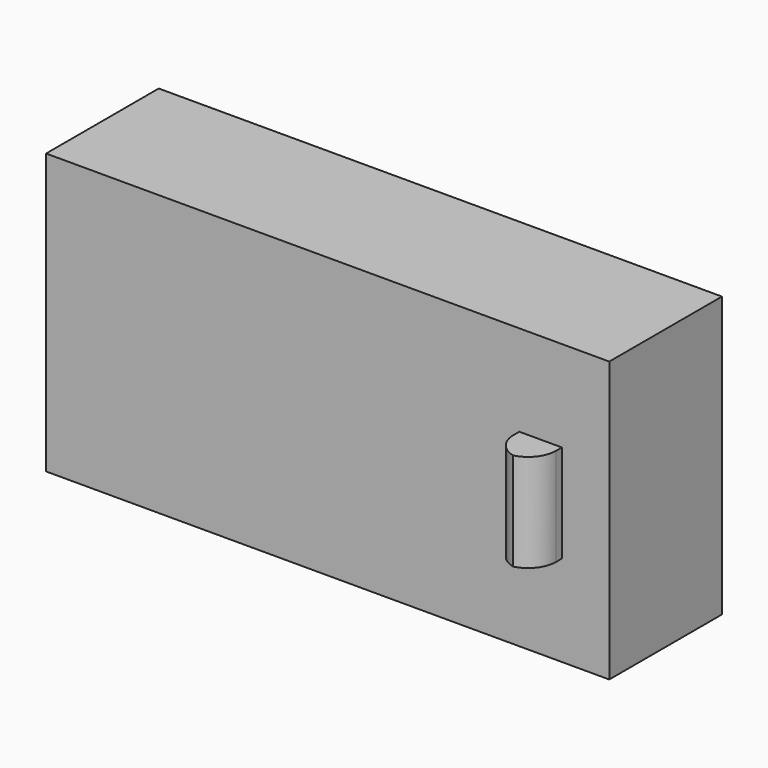
from build123d import *

# Parameters (mm, degrees)
F0_W        = 7.6837688684
F0_H        = 17.6492575556
F1_DEPTH    = 31.75
F0_W_2      = 101.6
F0_H_2      = 50.4952
F2_DEPTH    = 25.4
F3_T1_DEPTH = 43.0492575556


# Not quite as in the source:
# - a fillet or chamfer that OpenCascade refuses, or shapes differently, is made with other operations: its cross-section is extruded or revolved along the edge and cut away or added


with BuildPart() as f1:
    # F0 (on Front) → F1 (new body)
    with BuildSketch(Plane.XZ):
        with Locations((38.4069420397, 0)):
            Rectangle(F0_W, F0_H)
    extrude(amount=F1_DEPTH)

    # F0 (on Front) → F2 (join)
    with BuildSketch(Plane.XZ):
        Rectangle(F0_W_2, F0_H_2)
        with Locations((38.4069420397, 0)):
            Rectangle(F0_W, F0_H, mode=Mode.SUBTRACT)
    extrude(amount=F2_DEPTH)

    # F3: fillet of radius 5.08 on 2 edges, made by hand

    # F3_s2 → F3_t1 (cut)
    with BuildSketch(Plane.XY.offset(-21.5246287778)):
        with BuildLine():
            ThreePointArc((42.248826474, -26.67), (40.7609289224, -30.2621024484), (37.168826474, -31.75))
            Line((37.168826474, -31.75), (42.248826474, -31.75))
            Line((42.248826474, -31.75), (42.248826474, -26.67))
        make_face()
        with BuildLine():
            ThreePointArc((39.6450576055, -31.75), (36.0529551571, -30.2621024484), (34.5650576055, -26.67))
            Line((34.5650576055, -26.67), (34.5650576055, -31.75))
            Line((34.5650576055, -31.75), (39.6450576055, -31.75))
        make_face()
    extrude(amount=F3_T1_DEPTH, mode=Mode.SUBTRACT)


solid = f1.part
